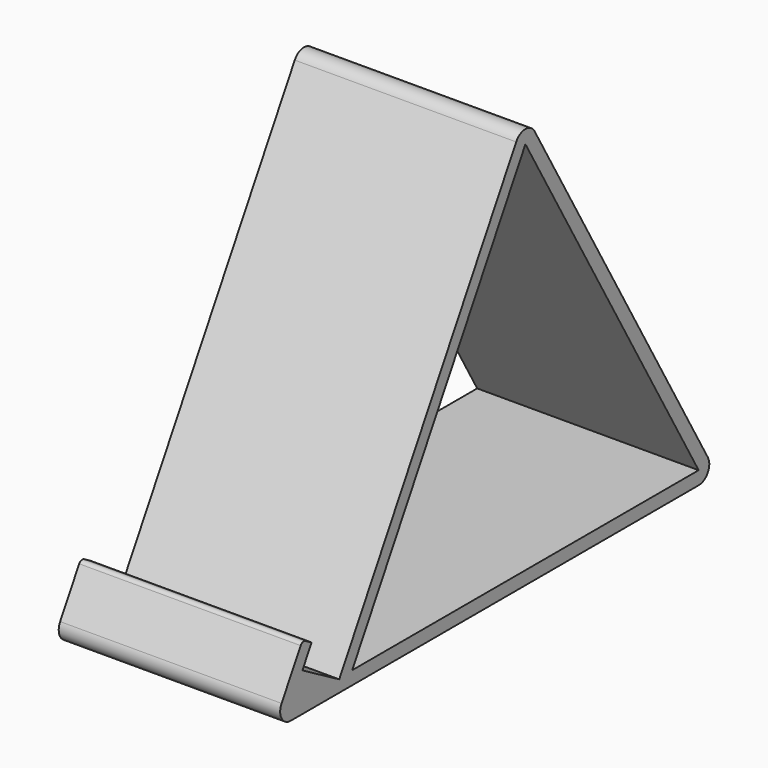
from build123d import *

# Parameters (mm, degrees)
F1_DEPTH = 50
F2_T     = 3
F4_DEPTH = 50


# Not quite as in the source:
# - a shell that OpenCascade refuses in one call is made with other operations: the cavity is built on its own and cut out


with BuildPart() as f1:
    # F0 (on Right) → F1 (new body)
    with BuildSketch(Plane.YZ):
        with BuildLine():
            Line((-2.5980762114, 57.9554029985), (-54.0879656003, -31.2277014993))
            Line((-54.0879656003, -31.2277014993), (48.8918131776, -31.2277014993))
            ThreePointArc((48.8918131776, -31.2277014993), (51.4898893889, -29.7277014993), (51.4898893889, -26.7277014993))
            Line((51.4898893889, -26.7277014993), (2.5980762114, 57.9554029985))
            ThreePointArc((2.5980762114, 57.9554029985), (0, 59.4554029985), (-2.5980762114, 57.9554029985))
        make_face()
    extrude(amount=F1_DEPTH)

    # F2: shell of thickness 3, made by hand


with BuildPart() as f2_core1:
    # F2_t2: copy of F1
    add(f1.part)

    # the walls: a layer under each face that stays
    f2_faces = [f2_core1.faces().sort_by_distance(p)[0] for p in [
        (25, -28.3430209058, 13.3638507496),
        (25, -2.5980762114, -31.2277014993),
        (25, 27.0439828001, 15.6138507496),
    ]]
    thicken(f2_faces, amount=-F2_T, mode=Mode.SUBTRACT)


with BuildPart() as f1_1:
    add(f1.part)

    # what is left inside the walls is the cavity
    f2_cavity = [f2_core1.part.solids().sort_by_distance(p)[0] for p in [
        (33.333333, -24.419926, 14.098851),
    ]]
    add(f2_cavity, mode=Mode.SUBTRACT)

    # F3 (on Right) → F4 (join)
    with BuildSketch(Plane.YZ):
        with BuildLine():
            Line((-54.0879656003, -31.2277014993), (-52.5466056017, -28.5579876689))
            Line((-52.5466056017, -28.5579876689), (-62.9389104471, -22.5579876689))
            Line((-62.9389104471, -22.5579876689), (-60.3408342357, -18.0579876689))
            Line((-60.3408342357, -18.0579876689), (-62.0728850433, -17.0579876689))
            ThreePointArc((-62.0728850433, -17.0579876689), (-62.8317040884, -16.9580872464), (-63.4389104471, -17.4240130727))
            Line((-63.4389104471, -17.4240130727), (-68.8103974646, -26.7277014993))
            ThreePointArc((-68.8103974646, -26.7277014993), (-68.8103974646, -29.7277014993), (-66.2123212533, -31.2277014993))
            Line((-66.2123212533, -31.2277014993), (-54.0879656003, -31.2277014993))
        make_face()
    extrude(amount=F4_DEPTH)


solid = f1_1.part
